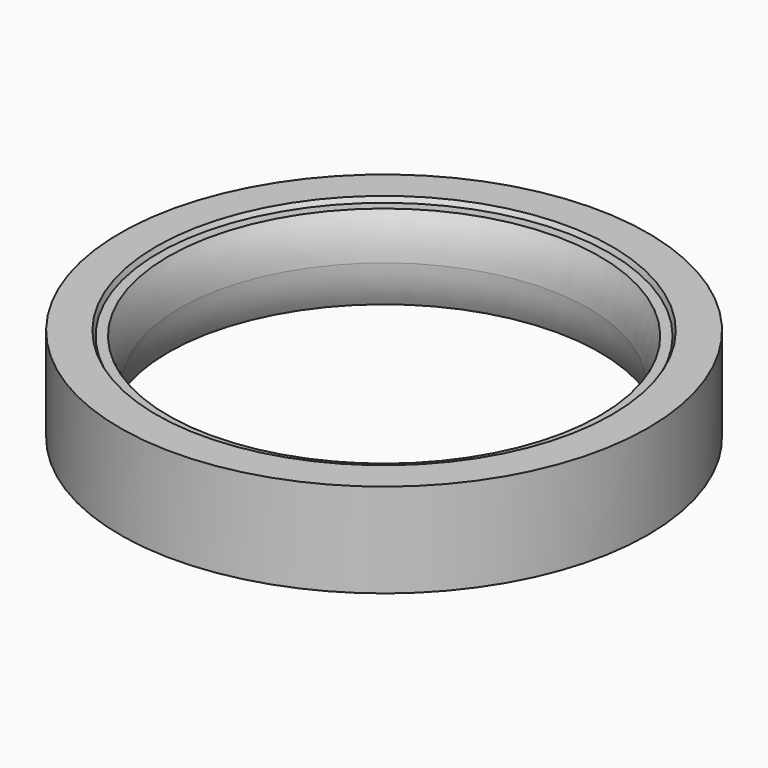
from build123d import *


# Not quite as in the source:
# - a feature of the source that left no trace in its solid (it failed there, or was rolled back) is left out


with BuildPart() as f1:
    # F0 (on Front) → F1 (revolve)
    with BuildSketch(Plane.XZ):
        with BuildLine():
            Line((10.95, 1.95), (9.45, 1.95))
            ThreePointArc((9.45, 1.95), (8.95, 0), (9.45, -1.95))
            Line((9.45, -1.95), (10.95, -1.95))
            Line((10.95, -1.95), (10.95, 1.95))
        make_face()
    revolve(axis=Axis((0, 0, 0.975), (0, 0, 1)))


with BuildPart() as f4:
    # F3 (on face) → F4 (revolve)
    with BuildSketch(Plane.XZ):
        with BuildLine():
            Line((8.9473315702, -1.75), (9.3473315702, -1.75))
            ThreePointArc((9.3473315702, -1.75), (8.95, 0), (9.3473315702, 1.75))
            Line((9.3473315702, 1.75), (8.9473315702, 1.75))
            ThreePointArc((8.9473315702, 1.75), (8.6136023479, 0.9031342001), (8.5, 0))
            ThreePointArc((8.5, 0), (8.6136023479, -0.9031342001), (8.9473315702, -1.75))
        make_face()
    revolve(axis=Axis((0, 0, 0.975), (0, 0, 1)))


solid = Compound([f1.part, f4.part])
